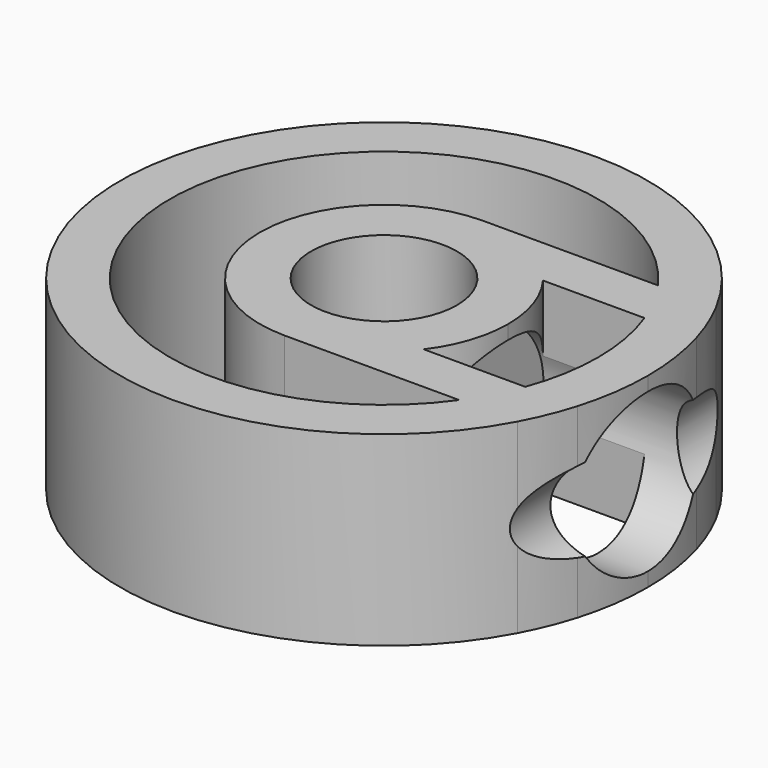
from build123d import *

# Parameters (mm, degrees)
F1_DEPTH      = 30
F3_START      = 15.5
F2_R          = 12.75
F3_DEPTH      = 30
F4_R          = 7.5
F5_DEPTH      = 25
F5_DEPTH_BACK = 25
F6_R          = 11.75
F7_DEPTH      = 28
F8_R          = 1.55
F9_DEPTH      = 10
F14_R         = 2.1
F15_DEPTH     = 2
F16_R         = 1.5
F17_DEPTH     = 2.4
F18_R         = 1


# Not quite as in the source:
# - a fillet or chamfer that OpenCascade refuses, or shapes differently, is made with other operations: its cross-section is extruded or revolved along the edge and cut away or added


with BuildPart() as f1:
    # F0 (on Top) → F1 (new body)
    with BuildSketch(Plane.XY):
        with BuildLine():
            Line((7.7707002638, -18.4286792096), (7.7707002638, 18.4286792096))
            ThreePointArc((7.7707002638, 18.4286792096), (3.963988888, 19.6032342254), (0, 20))
            ThreePointArc((0, 20), (-20, 0), (0, -20))
            ThreePointArc((0, -20), (3.963988888, -19.6032342254), (7.7707002638, -18.4286792096))
        make_face()
        with BuildLine():
            Line((7.7707002638, 18.4286792096), (7.7707002638, 20))
            Line((7.7707002638, 20), (0, 20))
            ThreePointArc((0, 20), (3.963988888, 19.6032342254), (7.7707002638, 18.4286792096))
        make_face()
        with BuildLine():
            Line((0, -20), (7.7707002638, -20))
            Line((7.7707002638, -20), (7.7707002638, -18.4286792096))
            ThreePointArc((7.7707002638, -18.4286792096), (3.963988888, -19.6032342254), (0, -20))
        make_face()
        with BuildLine():
            Line((15.7707002638, 12), (16, 12))
            ThreePointArc((16, 12), (12.3123323076, 15.7609159996), (7.7707002638, 18.4286792096))
            Line((7.7707002638, 18.4286792096), (7.7707002638, -18.4286792096))
            ThreePointArc((7.7707002638, -18.4286792096), (12.3123323076, -15.7609159996), (16, -12))
            Line((16, -12), (15.7707002638, -12))
            Line((15.7707002638, -12), (15.7707002638, 12))
        make_face()
        with BuildLine():
            ThreePointArc((28.1113855937, -20), (30.4920884675, -16.1394715183), (32.3457879793, -12))
            Line((32.3457879793, -12), (16, -12))
            ThreePointArc((16, -12), (12.3123323076, -15.7609159996), (7.7707002638, -18.4286792096))
            Line((7.7707002638, -18.4286792096), (7.7707002638, -20))
            Line((7.7707002638, -20), (28.1113855937, -20))
        make_face()
        with BuildLine():
            ThreePointArc((20, 0), (18.973665961, 6.3245553203), (16, 12))
            Line((16, 12), (15.7707002638, 12))
            Line((15.7707002638, 12), (15.7707002638, -12))
            Line((15.7707002638, -12), (16, -12))
            ThreePointArc((16, -12), (18.973665961, -6.3245553203), (20, 0))
        make_face()
        with BuildLine():
            Line((16, 12), (32.3457879793, 12))
            ThreePointArc((32.3457879793, 12), (30.4920884675, 16.1394715183), (28.1113855937, 20))
            Line((28.1113855937, 20), (7.7707002638, 20))
            Line((7.7707002638, 20), (7.7707002638, 18.4286792096))
            ThreePointArc((7.7707002638, 18.4286792096), (12.3123323076, 15.7609159996), (16, 12))
        make_face()
        with BuildLine():
            Line((32.3457879793, 12), (40.7707002638, 12))
            ThreePointArc((40.7707002638, 12), (39.3392377906, 16.0833569274), (37.5, 20))
            Line((37.5, 20), (28.1113855937, 20))
            ThreePointArc((28.1113855937, 20), (30.4920884675, 16.1394715183), (32.3457879793, 12))
        make_face()
        with BuildLine():
            Line((28.1113855937, 20), (37.5, 20))
            ThreePointArc((37.5, 20), (-42.5, 0), (37.5, -20))
            Line((37.5, -20), (28.1113855937, -20))
            ThreePointArc((28.1113855937, -20), (-34.5, 0), (28.1113855937, 20))
        make_face()
        with BuildLine():
            ThreePointArc((37.5, -20), (39.3392377906, -16.0833569274), (40.7707002638, -12))
            Line((40.7707002638, -12), (32.3457879793, -12))
            ThreePointArc((32.3457879793, -12), (30.4920884675, -16.1394715183), (28.1113855937, -20))
            Line((28.1113855937, -20), (37.5, -20))
        make_face()
        with BuildLine():
            Line((40.7707002638, -12), (40.7707002638, 12))
            Line((40.7707002638, 12), (32.3457879793, 12))
            ThreePointArc((32.3457879793, 12), (33.9571766, 6.0959131685), (34.5, 0))
            ThreePointArc((34.5, 0), (33.9571766, -6.0959131685), (32.3457879793, -12))
            Line((32.3457879793, -12), (40.7707002638, -12))
        make_face()
        with BuildLine():
            ThreePointArc((40.7707002638, -12), (42.0654535291, -6.0619814743), (42.5, 0))
            ThreePointArc((42.5, 0), (42.0654535291, 6.0619814743), (40.7707002638, 12))
            Line((40.7707002638, 12), (40.7707002638, -12))
        make_face()
    extrude(amount=F1_DEPTH)

    # F2 (on Right) → F3 (cut)
    with BuildSketch(Plane.YZ.offset(F3_START)):
        with Locations((0, 15)):
            Circle(F2_R)
    extrude(amount=F3_DEPTH, mode=Mode.SUBTRACT)

    # F4 (on Front) → F5 (cut, two sides)
    with BuildSketch(Plane.XZ) as f5_sk:
        with Locations((44.5, 15)):
            Circle(F4_R)
    extrude(amount=-F5_DEPTH, mode=Mode.SUBTRACT)
    extrude(f5_sk.sketch, amount=F5_DEPTH_BACK, mode=Mode.SUBTRACT)

    # F6 (on face) → F7 (cut)
    with BuildSketch(Plane.XY.offset(30)):
        Circle(F6_R)
    extrude(amount=-F7_DEPTH, mode=Mode.SUBTRACT)

    # F8 (on face) → F9 (cut)
    with BuildSketch(Plane.YZ.offset(15.5)):
        with Locations((0, 15)):
            Circle(F8_R)
    extrude(amount=-F9_DEPTH, mode=Mode.SUBTRACT)

    # F10 (on Front) → F11 (revolve)
    with BuildSketch(Plane.XZ):
        Polygon((0, 4.4), (0, 2), (4.65, 2), (2.1, 4.4), align=None)
    revolve(axis=Axis((0, 0, 6.6192487312), (0, 0, 1)))

    # F12 (on Front) → F13 (revolve, cut)
    with BuildSketch(Plane.XZ):
        with BuildLine():
            ThreePointArc((0, -9.9), (4.7022600949, -7.9522600949), (6.65, -3.25))
            ThreePointArc((6.65, -3.25), (4.7022600949, 1.4522600949), (0, 3.4))
            Line((0, 3.4), (0, -9.9))
        make_face()
    revolve(axis=Axis((0, 0, -3.25), (0, 0, -1)), mode=Mode.SUBTRACT)

    # F14 (on face) → F15 (join)
    with BuildSketch(Plane.XY.offset(4.4)):
        Circle(F14_R)
    extrude(amount=F15_DEPTH)

    # F16 (on face) → F17 (cut)
    with BuildSketch(Plane.XY.offset(6.4)):
        Circle(F16_R)
    extrude(amount=-F17_DEPTH, mode=Mode.SUBTRACT)

    # F18
    f18_edges = [f1.edges().sort_by_distance(p)[0] for p in [
        (-2.1, 0, 4.4),
        (-4.65, 0, 2),
    ]]
    fillet(f18_edges, radius=F18_R)

    # F19: chamfer of 0.4 on 1 edges, made by hand

    # F19_s1 → F19_t2 (revolve, cut)
    with BuildSketch(Plane.XZ):
        with BuildLine():
            Line((6.2028339317, -0.0077040086), (5.5986981628, 0.3241952337))
            Line((5.5986981628, 0.3241952337), (5.5919460169, 0.3199047179))
            ThreePointArc((5.5919460169, 0.3199047179), (5.6990064099, 0.1613765462), (5.7947443643, -0.0039097744))
            Line((5.7947443643, -0.0039097744), (5.8017238817, -0.008))
            ThreePointArc((5.8017238817, -0.008), (6.0022789067, -0.008), (6.2028339317, -0.0157040086))
            Line((6.2028339317, -0.0157040086), (6.2028339317, -0.0077040086))
        make_face()
    revolve(axis=Axis((0, 0, 0), (0, 0, 1)), mode=Mode.SUBTRACT)


solid = f1.part
